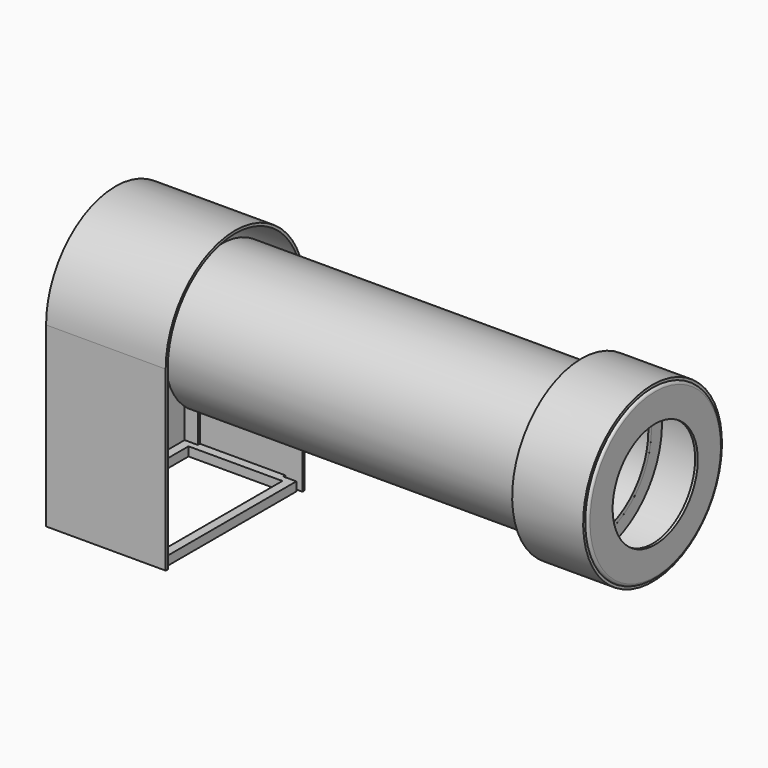
from build123d import *

# Parameters (mm, degrees)
F1_R         = 27
F1_R_2       = 25.5
F2_DEPTH     = 141.8
F4_W         = 5
F4_H         = 5
F8_R         = 1
F10_W        = 1
F10_H        = 67.5
F11_DEPTH    = 45.5
F12_W        = 42.5
F12_H        = 64
F12_W_2      = 35.7
F12_H_2      = 57.2
F13_DEPTH    = 3.4
F14_R        = 10.125
F14_W        = 64
F14_H        = 3.4
F15_DEPTH    = 1
F16_W        = 5
F16_H        = 1
F17_DEPTH    = 25
F18_W        = 5
F18_H        = 1
F20_T1_DEPTH = 72.5
F20_T3_DEPTH = 74
F20_T6_ANGLE = 180


# Not quite as in the source:
# - a fillet or chamfer that OpenCascade refuses, or shapes differently, is made with other operations: its cross-section is extruded or revolved along the edge and cut away or added


with BuildPart() as f2:
    # F1 (on Right) → F2 (new body)
    with BuildSketch(Plane.YZ):
        Circle(F1_R)
        Circle(F1_R_2, mode=Mode.SUBTRACT)
    extrude(amount=F2_DEPTH)


with BuildPart() as f5:
    # F4 (on Front) → F5 (revolve)
    with BuildSketch(Plane.XZ):
        with Locations((139.3, 29.5)):
            Rectangle(F4_W, F4_H)
    revolve(axis=Axis((153.0082076788, 0, 0), (-1, 0, 0)))


with BuildPart() as f6:
    # F4 (on Front) → F6 (revolve)
    with BuildSketch(Plane.XZ):
        Polygon((136.8, 33), (136.8, 32), (141.8, 32), (158.8, 32), (163.8, 32), (163.8, 33), align=None)
    revolve(axis=Axis((153.0082076788, 0, 0), (-1, 0, 0)))


with BuildPart() as f7:
    # F4 (on Front) → F7 (revolve)
    with BuildSketch(Plane.XZ):
        Polygon((163.8, 32), (158.8, 32), (158.8, 31), (163.8, 31), (163.8, 20.25), (164.8, 20.25), (164.8, 32), align=None)
    revolve(axis=Axis((153.0082076788, 0, 0), (-1, 0, 0)))

    # F8
    f8_edges = [f7.edges().sort_by_distance(p)[0] for p in [
        (164.8, 0, -32),
    ]]
    fillet(f8_edges, radius=F8_R)


with BuildPart() as f11:
    # F10 (on offset) → F11 (new body)
    with BuildSketch(Plane(origin=(5, 0, 0), x_dir=(0, -1, 0), z_dir=(-1, 0, 0))):
        with BuildLine():
            ThreePointArc((-32, 0), (0, 32), (32, 0))
            Line((32, 0), (33, 0))
            ThreePointArc((33, 0), (0, 33), (-33, 0))
            Line((-33, 0), (-32, 0))
        make_face()
        with Locations((32.5, -33.75)):
            Rectangle(F10_W, F10_H)
        with Locations((-32.5, -33.75)):
            Rectangle(F10_W, F10_H)
    extrude(amount=F11_DEPTH)


with BuildPart() as f13:
    # F12 (on face) → F13 (new body)
    with BuildSketch(Plane(origin=(0, 0, -67.5), x_dir=(1, 0, 0), z_dir=(0, 0, -1))):
        with Locations((-17.75, 0)):
            Rectangle(F12_W, F12_H)
        with Locations((-17.75, 0)):
            Rectangle(F12_W_2, F12_H_2, mode=Mode.SUBTRACT)
    extrude(amount=-F13_DEPTH)

    # F16 (on face) → F17 (cut)
    with BuildSketch(Plane(origin=(0, 0, -67.5), x_dir=(1, 0, 0), z_dir=(0, 0, -1))):
        with Locations((-36.5, 31.5)):
            Rectangle(F16_W, F16_H)
        with Locations((1, 31.5)):
            Rectangle(F16_W, F16_H)
        with Locations((-36.5, -31.5)):
            Rectangle(F16_W, F16_H)
        with Locations((1, -31.5)):
            Rectangle(F16_W, F16_H)
    extrude(amount=-F17_DEPTH, mode=Mode.SUBTRACT)


with BuildPart() as f15:
    # F14 (on face) → F15 (new body)
    with BuildSketch(Plane(origin=(-39, 0, 0), x_dir=(0, -1, 0), z_dir=(-1, 0, 0))):
        with BuildLine():
            Line((32, -64.1), (32, 0))
            ThreePointArc((32, 0), (0, 32), (-32, 0))
            Line((-32, 0), (-32, -64.1))
            Line((-32, -64.1), (32, -64.1))
        make_face()
        with Locations((0, -10.125)):
            Circle(F14_R, mode=Mode.SUBTRACT)
        with Locations((0, -65.8)):
            Rectangle(F14_W, F14_H)
    extrude(amount=F15_DEPTH)

    # F19: sweep along a path in F19_path
    with BuildLine(Plane(origin=(-39, -32, 0), x_dir=(0, 0, 1), z_dir=(1, 0, 0))) as f19_path:
        Line((-67.5, 0), (0, 0))
        ThreePointArc((0, 0), (32, -32), (0, -64))
        Line((0, -64), (-67.5, -64))
    # F18 (on face) → F19 (sweep)
    with BuildSketch(Plane(origin=(0, 0, -67.5), x_dir=(1, 0, 0), z_dir=(0, 0, -1))):
        with Locations((-36.5, 31.5)):
            Rectangle(F18_W, F18_H)
    sweep(path=f19_path.line)

    # F20: fillet of radius 2 on 5 edges, made by hand

    # F20_s2 → F20_t1 (cut)
    with BuildSketch(Plane.XY.offset(-72.5)):
        with BuildLine():
            ThreePointArc((-38, 32), (-39.4142135624, 31.4142135624), (-40, 30))
            Line((-40, 30), (-40, 32))
            Line((-40, 32), (-38, 32))
        make_face()
        with BuildLine():
            ThreePointArc((-38, -32), (-39.4142135624, -31.4142135624), (-40, -30))
            Line((-40, -30), (-40, -32))
            Line((-40, -32), (-38, -32))
        make_face()
    extrude(amount=F20_T1_DEPTH, mode=Mode.SUBTRACT)

    # F20_s4 → F20_t3 (cut)
    with BuildSketch(Plane.XZ.offset(-37)):
        with BuildLine():
            ThreePointArc((-38, -67.5), (-39.4142135624, -66.9142135624), (-40, -65.5))
            Line((-40, -65.5), (-40, -67.5))
            Line((-40, -67.5), (-38, -67.5))
        make_face()
    extrude(amount=F20_T3_DEPTH, mode=Mode.SUBTRACT)

    # F20_s5 → F20_t6 (revolve, cut)
    with BuildSketch(Plane.XY):
        with BuildLine():
            ThreePointArc((-40, -30), (-39.4142135624, -31.4142135624), (-38, -32))
            Line((-38, -32), (-40, -32))
            Line((-40, -32), (-40, -30))
        make_face()
    revolve(axis=Axis((-40, 0, 0), (-1, 0, 0)), revolution_arc=F20_T6_ANGLE, mode=Mode.SUBTRACT)

    # F20_s7 → F20_t8 (revolve, cut)
    with BuildSketch(Plane.XY.offset(-10.125)):
        with BuildLine():
            ThreePointArc((-39, -10.125), (-39.7320508076, -10.8570508076), (-40, -11.8570508076))
            Line((-40, -11.8570508076), (-40, -10.125))
            Line((-40, -10.125), (-39, -10.125))
        make_face()
    revolve(axis=Axis((-40, 0, -10.125), (-1, 0, 0)), mode=Mode.SUBTRACT)


solid = Compound([f2.part, f5.part, f6.part, f7.part, f11.part, f13.part, f15.part])
